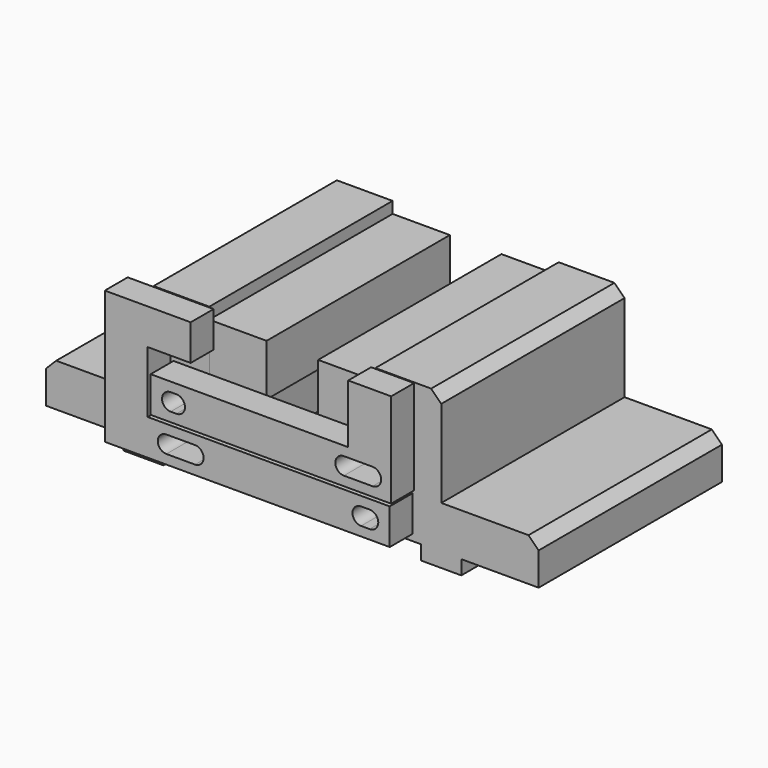
from build123d import *

# Parameters (mm, degrees)
F1_DEPTH  = 40
F2_W      = 3
F2_H      = 18
F3_W      = 3
F3_H      = 18
F4_DEPTH  = 80
F5_W      = 15
F5_H      = 20.5
F6_DEPTH  = 10
F7_DEPTH  = 20
F10_DEPTH = 20
F9_W      = 15
F9_H      = 12.5
F11_DEPTH = 10
F12_W     = 20
F12_H     = 18
F13_DEPTH = 80
F14_R     = 3
F15_DEPTH = 20


# Not quite as in the source:
# - a feature names something its author has since deleted; it is built from what else it names


with BuildPart() as f1:
    # F0 (on Front) → F1 (new body, symmetric)
    with BuildSketch(Plane.XZ):
        Polygon((-45, 0), (-26, 0), (-26, 45), (-29, 45), (-29, 49), (-48.4644660941, 49), (-52, 45.4644660941), (-52, 15), (-82.4644660941, 15), (-86, 11.4644660941), (-86, 0), (-59, 0), (-59, -5), (-45, -5), align=None)
    extrude(amount=F1_DEPTH, both=True)


with BuildPart() as f1b:
    # F0 (on Front) → F1, piece 2 (new body, symmetric)
    with BuildSketch(Plane.XZ):
        Polygon((26, 0), (45, 0), (45, -5), (59, -5), (59, 0), (86, 0), (86, 11.4644660941), (82.4644660941, 15), (52, 15), (52, 45.4644660941), (48.4644660941, 49), (29, 49), (29, 45), (26, 45), align=None)
    extrude(amount=F1_DEPTH, both=True)


with BuildPart() as f4_tool:
    # F2 (on face) + F3 (on face) → F4 (new body)
    with BuildSketch(Plane(origin=(0, 40, 0), x_dir=(-1, 0, 0), z_dir=(0, 1, 0))):
        with Locations((-27.5, 36)):
            Rectangle(F2_W, F2_H)
    with BuildSketch(Plane(origin=(0, 40, 0), x_dir=(-1, 0, 0), z_dir=(0, 1, 0))):
        with Locations((27.5, 36)):
            Rectangle(F3_W, F3_H)
    extrude(amount=-F4_DEPTH)


with BuildPart() as f1_1:
    add(f1.part)

    # F4: cut by f4_tool
    add(f4_tool.part, mode=Mode.SUBTRACT)


with BuildPart() as f1b_1:
    add(f1b.part)

    # F4: cut by f4_tool
    add(f4_tool.part, mode=Mode.SUBTRACT)


with BuildPart() as f6:
    # F5 (on face) → F6 (new body)
    with BuildSketch(Plane.XZ.offset(40)):
        Polygon((-41.5, 28.25), (-41.5, 15.75), (42.5, 15.75), (42.5, 28.25), (27.5, 28.25), align=None)
        with BuildLine():
            Line((-34.5, 25), (-33.5, 25))
            Line((-33.5, 25), (-32.5, 25))
            ThreePointArc((-32.5, 25), (-29.5, 22), (-32.5, 19))
            Line((-32.5, 19), (-33.5, 19))
            Line((-33.5, 19), (-34.5, 19))
            ThreePointArc((-34.5, 19), (-37.5, 22), (-34.5, 25))
        make_face(mode=Mode.SUBTRACT)
        with BuildLine():
            Line((25.9999999072, 25), (33.5, 25))
            Line((33.5, 25), (36.0000002221, 25))
            ThreePointArc((36.0000002221, 25), (39.0000002221, 21.9999999354), (36.0000000928, 19))
            Line((36.0000000928, 19), (33.5, 19))
            Line((33.5, 19), (25.9999997779, 19))
            ThreePointArc((25.9999997779, 19), (23.0000002221, 22.0000000646), (25.9999999072, 25))
        make_face(mode=Mode.SUBTRACT)
        with Locations((35, 38.5)):
            Rectangle(F5_W, F5_H)
    extrude(amount=F6_DEPTH)


with BuildPart() as f7_tool:
    # F5 (on face) → F7 (new body)
    with BuildSketch(Plane.XZ.offset(40)):
        with BuildLine():
            ThreePointArc((-32.5, 19.1715728753), (-31.0505102572, 20.2679491924), (-30.5, 22))
            ThreePointArc((-30.5, 22), (-31.0505102572, 23.7320508076), (-32.5, 24.8284271247))
            Line((-32.5, 24.8284271247), (-32.5, 19.1715728753))
        make_face()
        with BuildLine():
            Line((-32.5, 19.1715728753), (-32.5, 24.8284271247))
            ThreePointArc((-32.5, 24.8284271247), (-32.9926940638, 24.956795679), (-33.5, 25))
            ThreePointArc((-33.5, 25), (-34.0073059362, 24.956795679), (-34.5, 24.8284271247))
            Line((-34.5, 24.8284271247), (-34.5, 19.1715728753))
            ThreePointArc((-34.5, 19.1715728753), (-34.0073059362, 19.043204321), (-33.5, 19))
            ThreePointArc((-33.5, 19), (-32.9926940638, 19.043204321), (-32.5, 19.1715728753))
        make_face()
        with BuildLine():
            Line((-34.5, 19.1715728753), (-34.5, 24.8284271247))
            ThreePointArc((-34.5, 24.8284271247), (-36.5, 22), (-34.5, 19.1715728753))
        make_face()
        with BuildLine():
            ThreePointArc((33.5, 19), (35.6213203436, 19.8786796564), (36.5, 22))
            ThreePointArc((36.5, 22), (35.6213203436, 24.1213203436), (33.5, 25))
            ThreePointArc((33.5, 25), (30.5, 22), (33.5, 19))
        make_face()
    extrude(amount=-F7_DEPTH)


with BuildPart() as f1_2:
    add(f1_1.part)

    # F7: cut by f7_tool
    add(f7_tool.part, mode=Mode.SUBTRACT)


with BuildPart() as f1b_2:
    add(f1b_1.part)

    # F7: cut by f7_tool
    add(f7_tool.part, mode=Mode.SUBTRACT)


with BuildPart() as f10_tool:
    # F9 (on face) → F10 (new body)
    with BuildSketch(Plane.XZ.offset(40)):
        with BuildLine():
            ThreePointArc((-33.5, 5.5), (-31.3786796564, 6.3786796564), (-30.5, 8.5))
            ThreePointArc((-30.5, 8.5), (-31.3786796564, 10.6213203436), (-33.5, 11.5))
            ThreePointArc((-33.5, 11.5), (-36.5, 8.5), (-33.5, 5.5))
        make_face()
        with BuildLine():
            Line((32, 5.9019237886), (32, 11.0980762114))
            ThreePointArc((32, 11.0980762114), (30.5, 8.5), (32, 5.9019237886))
        make_face()
        with BuildLine():
            Line((35, 5.9019237886), (35, 11.0980762114))
            ThreePointArc((35, 11.0980762114), (34.2764571353, 11.3977774789), (33.5, 11.5))
            ThreePointArc((33.5, 11.5), (32.7235428647, 11.3977774789), (32, 11.0980762114))
            Line((32, 11.0980762114), (32, 5.9019237886))
            ThreePointArc((32, 5.9019237886), (32.7235428647, 5.6022225211), (33.5, 5.5))
            ThreePointArc((33.5, 5.5), (34.2764571353, 5.6022225211), (35, 5.9019237886))
        make_face()
        with BuildLine():
            ThreePointArc((35, 5.9019237886), (36.0980762114, 7), (36.5, 8.5))
            ThreePointArc((36.5, 8.5), (36.0980762114, 10), (35, 11.0980762114))
            Line((35, 11.0980762114), (35, 5.9019237886))
        make_face()
    extrude(amount=-F10_DEPTH)


with BuildPart() as f1_3:
    add(f1_2.part)

    # F10: cut by f10_tool
    add(f10_tool.part, mode=Mode.SUBTRACT)


with BuildPart() as f1b_3:
    add(f1b_2.part)

    # F10: cut by f10_tool
    add(f10_tool.part, mode=Mode.SUBTRACT)


with BuildPart() as f11:
    # F9 (on face) → F11 (new body)
    with BuildSketch(Plane.XZ.offset(40)):
        Polygon((-57.5, 14.75), (-57.5, 2.25), (42, 2.25), (42, 14.75), (-42.5, 14.75), align=None)
        with BuildLine():
            Line((-36.0000002215, 11.5), (-33.5, 11.5))
            Line((-33.5, 11.5), (-26.0000002215, 11.5))
            ThreePointArc((-26.0000002215, 11.5), (-22.9999997785, 8.5000002215), (-25.9999997785, 5.5))
            Line((-25.9999997785, 5.5), (-33.5, 5.5))
            Line((-33.5, 5.5), (-35.9999997785, 5.5))
            ThreePointArc((-35.9999997785, 5.5), (-38.9999997785, 8.4999997785), (-36.0000002215, 11.5))
        make_face(mode=Mode.SUBTRACT)
        with BuildLine():
            Line((32, 11.5), (33.5, 11.5))
            Line((33.5, 11.5), (35, 11.5))
            ThreePointArc((35, 11.5), (38, 8.5), (35, 5.5))
            Line((35, 5.5), (33.5, 5.5))
            Line((33.5, 5.5), (32, 5.5))
            ThreePointArc((32, 5.5), (29, 8.5), (32, 11.5))
        make_face(mode=Mode.SUBTRACT)
        Polygon((-57.5, 48.75), (-57.5, 14.75), (-42.5, 14.75), (-42.5, 36.25), (-42.5, 48.75), align=None)
        with Locations((-35, 42.5)):
            Rectangle(F9_W, F9_H)
    extrude(amount=F11_DEPTH)


with BuildPart() as f13:
    # F12 (on face) → F13 (new body)
    with BuildSketch(Plane(origin=(0, 40, 0), x_dir=(-1, 0, 0), z_dir=(0, 1, 0))):
        with Locations((-19, 36)):
            Rectangle(F12_W, F12_H)
    extrude(amount=-F13_DEPTH)


with BuildPart() as f13b:
    # F12 (on face) → F13, piece 2 (new body)
    with BuildSketch(Plane(origin=(0, 40, 0), x_dir=(-1, 0, 0), z_dir=(0, 1, 0))):
        with Locations((19, 36)):
            Rectangle(F12_W, F12_H)
    extrude(amount=-F13_DEPTH)


with BuildPart() as f15_tool:
    # F14 (on face) → F15 (new body)
    with BuildSketch(Plane(origin=(0, 40, 0), x_dir=(-1, 0, 0), z_dir=(0, 1, 0))):
        with Locations((-33.5, 22)):
            Circle(F14_R)
        with Locations((-33.5, 8.5)):
            Circle(F14_R)
        with Locations((33.5, 8.5)):
            Circle(F14_R)
        with Locations((33.5, 22)):
            Circle(F14_R)
    extrude(amount=-F15_DEPTH)


with BuildPart() as f1_4:
    add(f1_3.part)

    # F15: cut by f15_tool
    add(f15_tool.part, mode=Mode.SUBTRACT)


with BuildPart() as f1b_4:
    add(f1b_3.part)

    # F15: cut by f15_tool
    add(f15_tool.part, mode=Mode.SUBTRACT)


solid = Compound([f6.part, f11.part, f13.part, f13b.part, f1_4.part, f1b_4.part])
